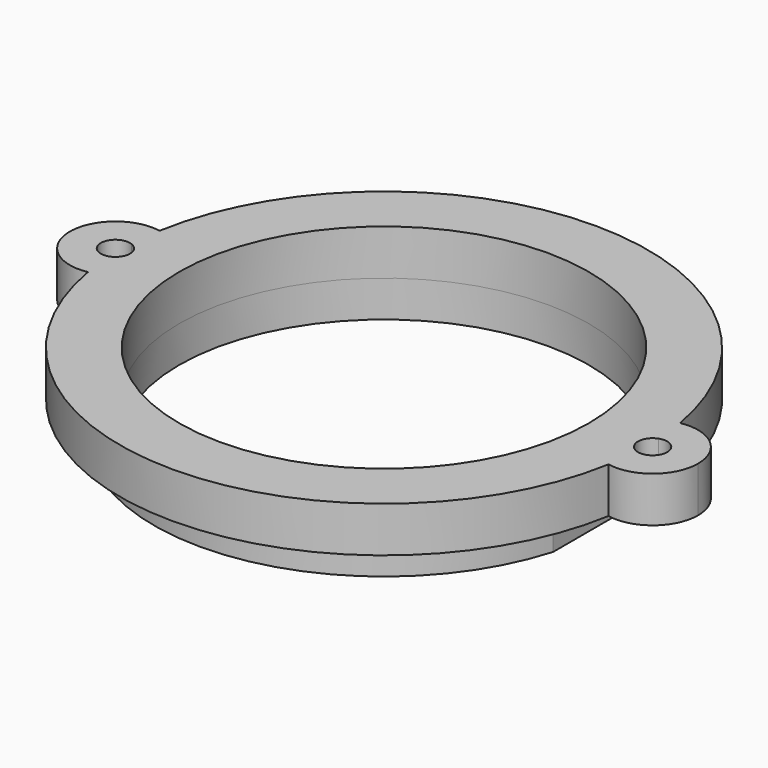
from build123d import *

# Parameters (mm, degrees)
F0_R     = 22.5
F1_DEPTH = 5
F2_DEPTH = 4


# Not quite as in the source:
# - a feature names something its author has since deleted; it is built from what else it names


with BuildPart() as f1:
    # F0 (on Top) → F1 (new body)
    with BuildSketch(Plane.XY):
        with BuildLine():
            ThreePointArc((28.5805084746, -4.9147263743), (24.5, 0), (28.5805084746, 4.9147263743))
            ThreePointArc((28.5805084746, 4.9147263743), (0, 29), (-28.5805084746, 4.9147263743))
            ThreePointArc((-28.5805084746, 4.9147263743), (-25.6530884058, 3.1939428903), (-24.5, 0))
            ThreePointArc((-24.5, 0), (-25.6530884058, -3.1939428903), (-28.5805084746, -4.9147263743))
            ThreePointArc((-28.5805084746, -4.9147263743), (0, -29), (28.5805084746, -4.9147263743))
        make_face()
        with BuildLine():
            ThreePointArc((-24.24, 7.07), (0, 25.25), (24.24, 7.07))
            Line((24.24, 7.07), (24.24, -7.07))
            ThreePointArc((24.24, -7.07), (0, -25.25), (-24.24, -7.07))
            Line((-24.24, -7.07), (-24.24, 7.07))
        make_face(mode=Mode.SUBTRACT)
        with BuildLine():
            Line((24.24, -7.07), (24.24, 7.07))
            ThreePointArc((24.24, 7.07), (0, 25.25), (-24.24, 7.07))
            Line((-24.24, 7.07), (-24.24, -7.07))
            ThreePointArc((-24.24, -7.07), (0, -25.25), (24.24, -7.07))
        make_face()
        Circle(F0_R, mode=Mode.SUBTRACT)
        with BuildLine():
            ThreePointArc((-28.9608474576, 1.506424421), (-28.8211040937, 3.2162025464), (-28.5805084746, 4.9147263743))
            ThreePointArc((-28.5805084746, 4.9147263743), (-34.5, 0), (-28.5805084746, -4.9147263743))
            ThreePointArc((-28.5805084746, -4.9147263743), (-28.8211040937, -3.2162025464), (-28.9608474576, -1.506424421))
            ThreePointArc((-28.9608474576, -1.506424421), (-31.1, 0), (-28.9608474576, 1.506424421))
        make_face()
        with BuildLine():
            ThreePointArc((28.5805084746, 4.9147263743), (28.8211040937, 3.2162025464), (28.9608474576, 1.506424421))
            ThreePointArc((28.9608474576, 1.506424421), (30.4212371932, 1.3081750777), (31.1, 0))
            ThreePointArc((31.1, 0), (30.4212371932, -1.3081750777), (28.9608474576, -1.506424421))
            ThreePointArc((28.9608474576, -1.506424421), (28.8211040937, -3.2162025464), (28.5805084746, -4.9147263743))
            ThreePointArc((28.5805084746, -4.9147263743), (32.6939428903, -3.8469115942), (34.5, 0))
            ThreePointArc((34.5, 0), (32.6939428903, 3.8469115942), (28.5805084746, 4.9147263743))
        make_face()
        with BuildLine():
            ThreePointArc((-24.5, 0), (-25.6530884058, 3.1939428903), (-28.5805084746, 4.9147263743))
            ThreePointArc((-28.5805084746, 4.9147263743), (-28.8211040937, 3.2162025464), (-28.9608474576, 1.506424421))
            ThreePointArc((-28.9608474576, 1.506424421), (-28.1918249223, 0.9212371932), (-27.9, 0))
            ThreePointArc((-27.9, 0), (-28.1918249223, -0.9212371932), (-28.9608474576, -1.506424421))
            ThreePointArc((-28.9608474576, -1.506424421), (-28.8211040937, -3.2162025464), (-28.5805084746, -4.9147263743))
            ThreePointArc((-28.5805084746, -4.9147263743), (-25.6530884058, -3.1939428903), (-24.5, 0))
        make_face()
        with BuildLine():
            ThreePointArc((28.9608474576, -1.506424421), (27.9, 0), (28.9608474576, 1.506424421))
            ThreePointArc((28.9608474576, 1.506424421), (28.8211040937, 3.2162025464), (28.5805084746, 4.9147263743))
            ThreePointArc((28.5805084746, 4.9147263743), (24.5, 0), (28.5805084746, -4.9147263743))
            ThreePointArc((28.5805084746, -4.9147263743), (28.8211040937, -3.2162025464), (28.9608474576, -1.506424421))
        make_face()
    extrude(amount=F1_DEPTH)

    # F0 (on Top) → F2 (join)
    with BuildSketch(Plane.XY):
        with BuildLine():
            Line((24.24, -7.07), (24.24, 7.07))
            ThreePointArc((24.24, 7.07), (0, 25.25), (-24.24, 7.07))
            Line((-24.24, 7.07), (-24.24, -7.07))
            ThreePointArc((-24.24, -7.07), (0, -25.25), (24.24, -7.07))
        make_face()
        Circle(F0_R, mode=Mode.SUBTRACT)
    extrude(amount=-F2_DEPTH)


solid = f1.part
